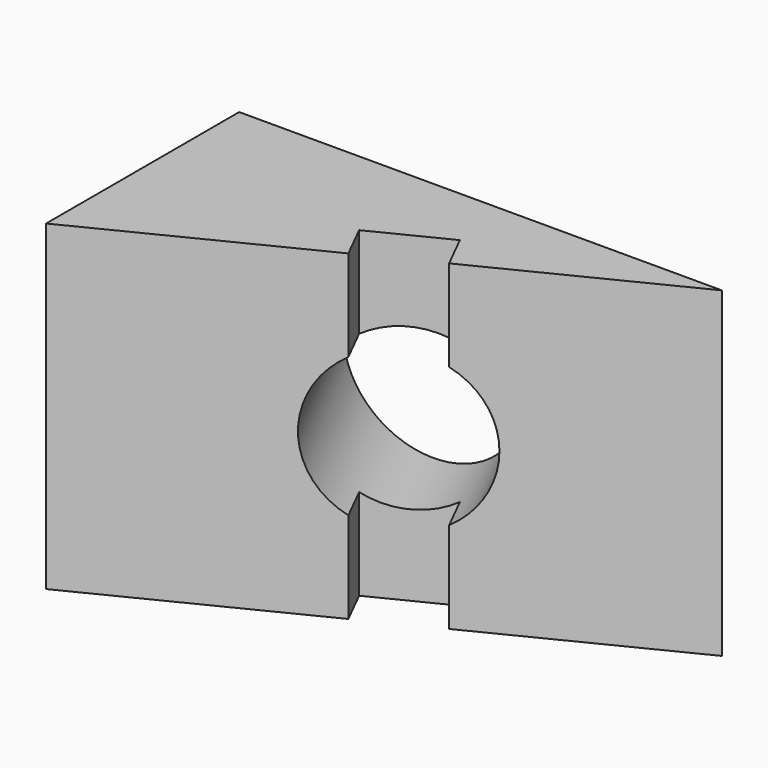
from build123d import *

# Parameters (mm, degrees)
F1_DEPTH = 101.6
F2_W     = 25.4
F2_H     = 101.6
F3_DEPTH = 12.7
F4_R     = 25.4
F5_DEPTH = 68.1563519542


# Not quite as in the source:
# - a feature names something its author has since deleted; it is built from what else it names


with BuildPart() as f1:
    # F0 (on Top) → F1 (new body)
    with BuildSketch(Plane.XY):
        Polygon((152.4, 0), (0, 0), (0, -76.2), align=None)
    extrude(amount=F1_DEPTH)

    # F2 (on face) → F3 (cut)
    with BuildSketch(Plane(origin=(30.48, -60.96, 0), x_dir=(0.894427191, 0.4472135955, 0), z_dir=(0.4472135955, -0.894427191, 0))):
        with Locations((54.8223240229, 50.8)):
            Rectangle(F2_W, F2_H)
    extrude(amount=-F3_DEPTH, mode=Mode.SUBTRACT)

    # F4 (on face) → F5 (cut, through all)
    with BuildSketch(Plane(origin=(30.48, -60.96, 0), x_dir=(0.894427191, 0.4472135955, 0), z_dir=(0.4472135955, -0.894427191, 0))):
        with Locations((54.8223240229, 50.8)):
            Circle(F4_R)
    extrude(amount=-F5_DEPTH, mode=Mode.SUBTRACT)


solid = f1.part
